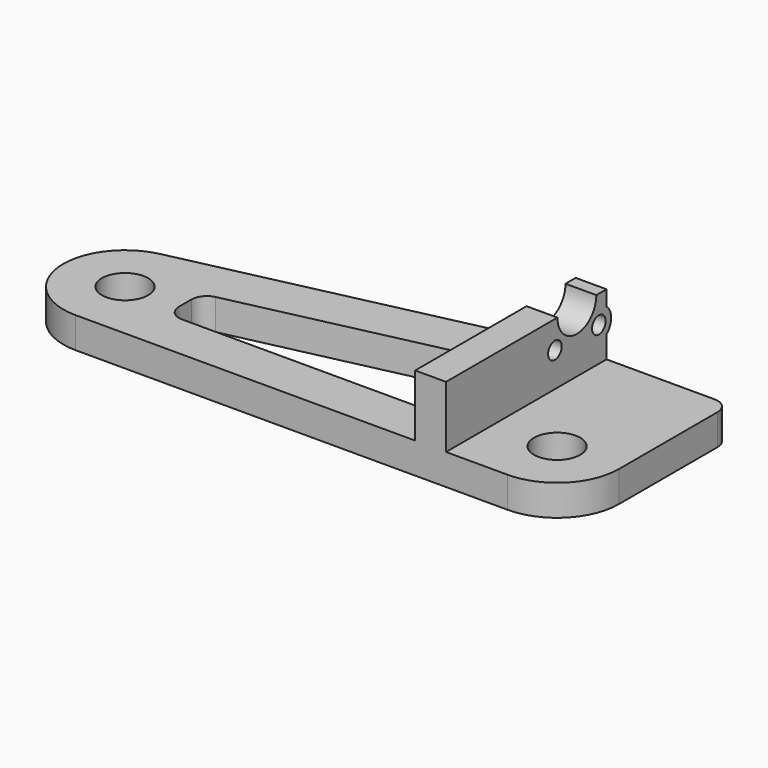
from build123d import *

# Parameters (mm, degrees)
F0_R      = 4.7625
F1_DEPTH  = 6.35
F2_R      = 12.69999
F3_W      = 6.35
F3_H      = 41.275
F4_DEPTH  = 12.7
F6_DEPTH  = 25.4
F7_R      = 3.175
F8_R      = 5.0038
F8_R_2    = 1.7526
F9_DEPTH  = 25.4
F11_DEPTH = 6.35


# Not quite as in the source:
# - a fillet or chamfer is up to 0.001 mm smaller than in the source, because OpenCascade refuses the exact size


with BuildPart() as f1:
    # F0 (on Top) → F1 (new body)
    with BuildSketch(Plane.XY):
        Polygon((-101.6, -12.7), (12.7, -12.7), (12.7, 28.575), (-19.05, 28.575), (-101.6, 10.1816951473), align=None)
        with Locations((-88.9, 0)):
            Circle(F0_R, mode=Mode.SUBTRACT)
        Circle(F0_R, mode=Mode.SUBTRACT)
    extrude(amount=F1_DEPTH)

    # F2 (radius 12.7 in the source; OpenCascade refuses exactly that, so slightly less here)
    f2_edges = [f1.edges().sort_by_distance(p)[0] for p in [
        (12.7, -12.7, 3.175),
        (-101.6, -12.7, 3.175),
        (-101.6, 10.181695, 3.175),
    ]]
    fillet(f2_edges, radius=F2_R)

    # F3 (on face) → F4 (join)
    with BuildSketch(Plane.XY.offset(6.35)):
        with Locations((-15.875, 7.9375)):
            Rectangle(F3_W, F3_H)
    extrude(amount=F4_DEPTH)

    # F5 (on face) → F6 (cut)
    with BuildSketch(Plane.XY.offset(6.35)):
        with BuildLine():
            Line((-19.05, 18.8164242334), (-75.3030020415, 6.2824615995))
            ThreePointArc((-75.3030020415, 6.2824615995), (-77.0896928651, 5.1694426385), (-77.7875, 3.1834566091))
            Line((-77.7875, 3.1834566091), (-77.7875, 0))
            ThreePointArc((-77.7875, 0), (-76.8575640303, -2.2450640303), (-74.6125, -3.175))
            Line((-74.6125, -3.175), (-19.05, -3.175))
            Line((-19.05, -3.175), (-19.05, 18.8164242334))
        make_face()
    extrude(amount=-F6_DEPTH, mode=Mode.SUBTRACT)

    # F7
    f7_edges = [f1.edges().sort_by_distance(p)[0] for p in [
        (12.7, 28.575, 3.175),
    ]]
    fillet(f7_edges, radius=F7_R)

    # F8 (on face) → F9 (cut)
    with BuildSketch(Plane.YZ.offset(-12.7)):
        with Locations((20.955, 19.05)):
            Circle(F8_R)
        with Locations((26.6065, 13.3985)):
            Circle(F8_R_2)
        with Locations((15.3035, 13.3985)):
            Circle(F8_R_2)
    extrude(amount=-F9_DEPTH, mode=Mode.SUBTRACT)

    # F10 (on face) → F11 (join)
    with BuildSketch(Plane.YZ.offset(-12.7)):
        with BuildLine():
            Line((28.575, 15.8896107462), (28.575, 10.9073892538))
            ThreePointArc((28.575, 10.9073892538), (29.7815, 13.3985), (28.575, 15.8896107462))
        make_face()
    extrude(amount=-F11_DEPTH)


solid = f1.part
